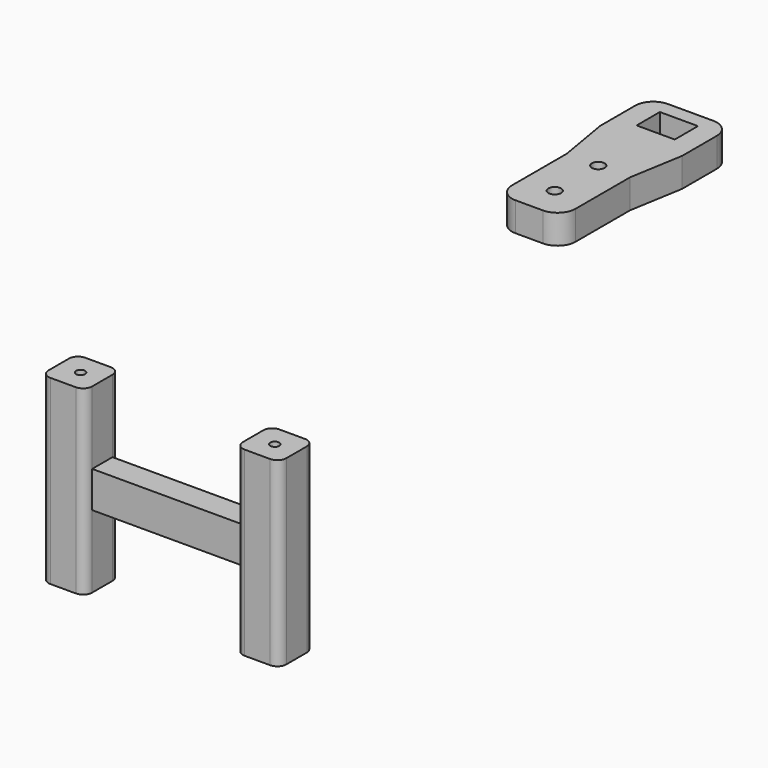
from build123d import *

# Parameters (mm, degrees)
F7_W      = 2.5
F7_H      = 17
F7_W_2    = 17.5
F7_W_3    = 10.5
F7_H_2    = 8
F7_R      = 1.75
F8_DEPTH  = 8
F9_R      = 5
F11_DEPTH = 6
F10_R     = 1.75
F12_DEPTH = 2
F15_DEPTH = 3.5
F16_DEPTH = 6
F18_D     = 2.5
F18_DEPTH = 12
F18_TIP   = 0.7510757738
F20_D     = 2.5
F20_DEPTH = 12
F20_TIP   = 0.7510757738
F21_R     = 2.49999


# Not quite as in the source:
# - a fillet or chamfer is up to 0.001 mm smaller than in the source, because OpenCascade refuses the exact size


with BuildPart() as f8:
    # F7 (on Top) → F8 (new body)
    with BuildSketch(Plane.XY):
        with Locations((10, 93.5713741661)):
            Rectangle(F7_W, F7_H)
        with Locations((0, 93.5713741661)):
            Rectangle(F7_W_2, F7_H)
        with Locations((0, 94.0713741661)):
            Rectangle(F7_W_3, F7_H_2, mode=Mode.SUBTRACT)
        with Locations((-10, 93.5713741661)):
            Rectangle(F7_W, F7_H)
        Polygon((-11.25, 85.0713741661), (-8.75, 70.3213741661), (-8.75, 85.0713741661), align=None)
        Polygon((-8.75, 46.5713741661), (8.75, 46.5713741661), (8.75, 70.3213741661), (8.75, 85.0713741661), (-8.75, 85.0713741661), (-8.75, 70.3213741661), align=None)
        with Locations((0, 55.3213741661)):
            Circle(F7_R, mode=Mode.SUBTRACT)
        with Locations((0, 70.3213741661)):
            Circle(F7_R, mode=Mode.SUBTRACT)
        Polygon((8.75, 85.0713741661), (8.75, 70.3213741661), (11.25, 85.0713741661), align=None)
    extrude(amount=-F8_DEPTH)

    # F9
    f9_edges = [f8.edges().sort_by_distance(p)[0] for p in [
        (11.25, 102.071374, -4),
        (8.75, 46.571374, -4),
        (-8.75, 46.571374, -4),
        (-11.25, 102.071374, -4),
    ]]
    fillet(f9_edges, radius=F9_R)

    # F10 (on face) → F11 (cut)
    with BuildSketch(Plane(origin=(0, 0, -8), x_dir=(1, 0, 0), z_dir=(0, 0, -1))):
        with BuildLine():
            Line((6.75, -57.3213741661), (4.8046514937, -57.3213741661))
            ThreePointArc((4.8046514937, -57.3213741661), (0, -60.5256681601), (-4.8046514937, -57.3213741661))
            Line((-4.8046514937, -57.3213741661), (-6.75, -57.3213741661))
            Line((-6.75, -57.3213741661), (-6.75, -68.3213741661))
            Line((-6.75, -68.3213741661), (-4.8046514937, -68.3213741661))
            ThreePointArc((-4.8046514937, -68.3213741661), (0, -65.1170801721), (4.8046514937, -68.3213741661))
            Line((4.8046514937, -68.3213741661), (6.75, -68.3213741661))
            Line((6.75, -68.3213741661), (6.75, -57.3213741661))
        make_face()
        with BuildLine():
            Line((-6.75, -53.3213741661), (-4.8046514937, -53.3213741661))
            ThreePointArc((-4.8046514937, -53.3213741661), (0, -50.1170801721), (4.8046514937, -53.3213741661))
            Line((4.8046514937, -53.3213741661), (6.75, -53.3213741661))
            Line((6.75, -53.3213741661), (6.75, -51.5713741661))
            ThreePointArc((6.75, -51.5713741661), (5.8713203436, -49.4500538226), (3.75, -48.5713741661))
            Line((3.75, -48.5713741661), (-3.75, -48.5713741661))
            ThreePointArc((-3.75, -48.5713741661), (-5.8713203436, -49.4500538226), (-6.75, -51.5713741661))
            Line((-6.75, -51.5713741661), (-6.75, -53.3213741661))
        make_face()
        with BuildLine():
            Line((9.25, -85.2396656064), (7.0604590779, -72.3213741661))
            Line((7.0604590779, -72.3213741661), (4.8046514937, -72.3213741661))
            ThreePointArc((4.8046514937, -72.3213741661), (0, -75.5256681601), (-4.8046514937, -72.3213741661))
            Line((-4.8046514937, -72.3213741661), (-7.0604590779, -72.3213741661))
            Line((-7.0604590779, -72.3213741661), (-9.25, -85.2396656064))
            Line((-9.25, -85.2396656064), (-9.25, -87.0713741661))
            Line((-9.25, -87.0713741661), (9.25, -87.0713741661))
            Line((9.25, -87.0713741661), (9.25, -85.2396656064))
        make_face()
    extrude(amount=-F11_DEPTH, mode=Mode.SUBTRACT)

    # F10 (on face) → F12 (cut)
    with BuildSketch(Plane(origin=(0, 0, -8), x_dir=(1, 0, 0), z_dir=(0, 0, -1))):
        Polygon((-2.0495934556, -57.3213741661), (2.0495934556, -57.3213741661), (3.204293994, -55.3213741661), (2.0495934556, -53.3213741661), (-2.0495934556, -53.3213741661), (-3.204293994, -55.3213741661), align=None)
        with Locations((0, -55.3213741661)):
            Circle(F10_R, mode=Mode.SUBTRACT)
        Polygon((-1.602146997, -58.0963741661), (1.602146997, -58.0963741661), (2.0495934556, -57.3213741661), (-2.0495934556, -57.3213741661), align=None)
        Polygon((-2.0495934556, -53.3213741661), (2.0495934556, -53.3213741661), (1.602146997, -52.5463741661), (-1.602146997, -52.5463741661), align=None)
        Polygon((2.0495934556, -72.3213741661), (-2.0495934556, -72.3213741661), (-1.602146997, -73.0963741661), (1.602146997, -73.0963741661), align=None)
        Polygon((3.204293994, -70.3213741661), (2.0495934556, -68.3213741661), (-2.0495934556, -68.3213741661), (-3.204293994, -70.3213741661), (-2.0495934556, -72.3213741661), (2.0495934556, -72.3213741661), align=None)
        with Locations((0, -70.3213741661)):
            Circle(F10_R, mode=Mode.SUBTRACT)
        Polygon((-2.0495934556, -68.3213741661), (2.0495934556, -68.3213741661), (1.602146997, -67.5463741661), (-1.602146997, -67.5463741661), align=None)
    extrude(amount=-F12_DEPTH, mode=Mode.SUBTRACT)


with BuildPart() as f15:
    # F14 (on line) → F15 (new body, symmetric)
    with BuildSketch(Plane(origin=(0, -74.4982883334, 0), x_dir=(-1, 0, 0), z_dir=(0, 1, 0))):
        Polygon((20.75, -20), (0, -20), (-20.75, -20), (-20.75, -30), (0, -30), (20.75, -30), align=None)
    extrude(amount=F15_DEPTH, both=True)

    # F14 (on line) → F16 (join, symmetric)
    with BuildSketch(Plane(origin=(0, -74.4982883334, 0), x_dir=(-1, 0, 0), z_dir=(0, 1, 0))):
        Polygon((20.75, 0), (20.75, -20), (20.75, -30), (20.75, -50), (32.75, -50), (32.75, -25), (32.75, 0), align=None)
        Polygon((-20.75, -30), (-20.75, -20), (-20.75, 0), (-32.75, 0), (-32.75, -25), (-32.75, -50), (-20.75, -50), align=None)
    extrude(amount=F16_DEPTH, both=True)

    # F18
    with Locations(Plane.XY):
        with Locations((-26.75, -74.4982883334), (26.75, -74.4982883334)):
            Hole(F18_D / 2, depth=F18_DEPTH)
            with Locations((0, 0, -(F18_DEPTH + F18_TIP / 2))):  # 118° drill point
                Cone(0, F18_D / 2, F18_TIP, mode=Mode.SUBTRACT)

    # F20
    with Locations(Plane(origin=(0, 0, -50), x_dir=(1, 0, 0), z_dir=(0, 0, -1))):
        with Locations((-26.75, 74.4982883334), (26.75, 74.4982883334)):
            Hole(F20_D / 2, depth=F20_DEPTH)
            with Locations((0, 0, -(F20_DEPTH + F20_TIP / 2))):  # 118° drill point
                Cone(0, F20_D / 2, F20_TIP, mode=Mode.SUBTRACT)

    # F21 (radius 2.5 in the source; OpenCascade refuses exactly that, so slightly less here)
    f21_edges = [f15.edges().sort_by_distance(p)[0] for p in [
        (-20.75, -80.498288, -25),
        (-20.75, -68.498288, -25),
        (-32.75, -80.498288, -25),
        (20.75, -80.498288, -25),
        (32.75, -80.498288, -25),
        (32.75, -68.498288, -25),
        (-32.75, -68.498288, -25),
        (20.75, -68.498288, -25),
    ]]
    fillet(f21_edges, radius=F21_R)


solid = Compound([f8.part, f15.part])
